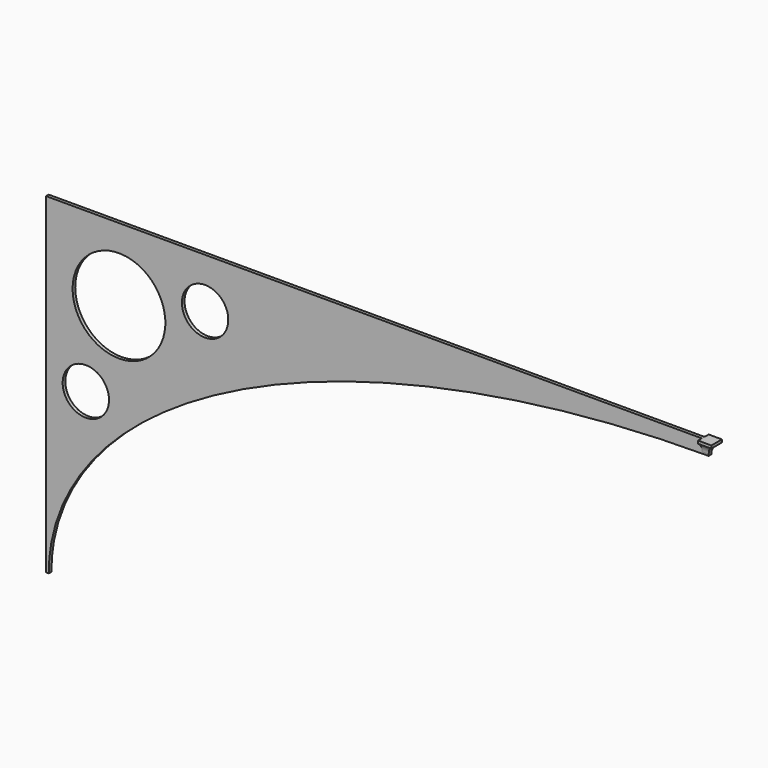
from build123d import *

# Parameters (mm, degrees)
F1_DEPTH     = 2.5
F3_D         = 70
F4_D         = 35
F5_W         = 5
F5_H         = 2.5
F6_DEPTH     = 2
F7_DEPTH     = 0.1
F8_T1_DEPTH  = 2.5
F8_T3_DEPTH  = 5
F8_T9_DEPTH  = 21.0404962177
F8_T14_DEPTH = 21.9443021397
F8_T22_DEPTH = 21.0404962177
F8_T27_DEPTH = 21.9443021397


# Not quite as in the source:
# - a fillet or chamfer that OpenCascade refuses, or shapes differently, is made with other operations: its cross-section is extruded or revolved along the edge and cut away or added


with BuildPart() as f1:
    # F0 (on Front) → F1 (new body)
    with BuildSketch(Plane.XZ):
        with BuildLine():
            Line((234.3109268695, 164.7265180945), (-265.6890731305, 164.7265180945))
            Line((-265.6890731305, 164.7265180945), (-265.6890731305, -85.2734819055))
            Line((-265.6890731305, -85.2734819055), (-263.6890731305, -85.2734819055))
            add(Edge.make_bspline(
                [(234.3109268695, 154.7265180945), (-263.6890731305, 154.7265180945), (-263.6890731305, -85.2734819055)],
                knots=[4.7123889804, 4.7123889804, 4.7123889804, 6.2831853072, 6.2831853072, 6.2831853072], degree=2, weights=[1, 0.7071067812, 1]))
            Line((234.3109268695, 154.7265180945), (234.3109268695, 164.7265180945))
        make_face()
    extrude(amount=F1_DEPTH)

    # F3 (through all)
    with Locations(Plane.XZ.offset(2.5)):
        with Locations((-210.6890731305, 109.7265180945)):
            Hole(F3_D / 2)

    # F4 (through all)
    with Locations(Plane.XZ.offset(2.5)):
        with Locations((-145.6890731305, 127.2265180945), (-235.6890731305, 44.7265180945)):
            Hole(F4_D / 2)

    # F5 (on face) → F6 (join)
    with BuildSketch(Plane.XY.offset(164.7265180945)):
        Polygon((239.3109268695, -6.25), (239.3109268695, 3.75), (229.3109268695, 3.75), (229.3109268695, 0), (234.3109268695, 0), (234.3109268695, -2.5), (229.3109268695, -2.5), (229.3109268695, -6.25), align=None)
        with Locations((231.8109268695, -1.25)):
            Rectangle(F5_W, F5_H)
    extrude(amount=-F6_DEPTH)

    # F5 (on face) → F7 (join)
    with BuildSketch(Plane.XY.offset(164.7265180945)):
        Polygon((239.3109268695, -6.25), (239.3109268695, 3.75), (229.3109268695, 3.75), (229.3109268695, 0), (234.3109268695, 0), (234.3109268695, -2.5), (229.3109268695, -2.5), (229.3109268695, -6.25), align=None)
        with Locations((231.8109268695, -1.25)):
            Rectangle(F5_W, F5_H)
    extrude(amount=F7_DEPTH)

    # F8: fillet of radius 8 on 3 edges, made by hand

    # F8_s2 → F8_t1 (join)
    with BuildSketch(Plane.XZ):
        with BuildLine():
            ThreePointArc((234.3109268695, 155.3103196074), (235.6776772888, 159.7824555624), (239.3109268695, 162.7265180945))
            Line((239.3109268695, 162.7265180945), (234.3109268695, 162.7265180945))
            Line((234.3109268695, 162.7265180945), (234.3109268695, 155.3103196074))
        make_face()
    extrude(amount=F8_T1_DEPTH)

    # F8_s4 → F8_t3 (join)
    with BuildSketch(Plane.YZ.offset(229.3109268695)):
        with BuildLine():
            ThreePointArc((-2.5, 155.9487972387), (-3.5, 159.8217805849), (-6.25, 162.7265180945))
            Line((-6.25, 162.7265180945), (-2.5, 162.7265180945))
            Line((-2.5, 162.7265180945), (-2.5, 155.9487972387))
        make_face()
        with BuildLine():
            ThreePointArc((3.75, 162.7265180945), (1, 159.8217805849), (0, 155.9487972387))
            Line((0, 155.9487972387), (0, 162.7265180945))
            Line((0, 162.7265180945), (3.75, 162.7265180945))
        make_face()
    extrude(amount=F8_T3_DEPTH)


with BuildPart() as f8_tool7:
    # F8_s8 → F8_t9 (new body)
    with BuildSketch(Plane.XZ.offset(21.0404962177)):
        with BuildLine():
            ThreePointArc((234.3109268695, 155.3103196074), (235.6776772888, 159.7824555624), (239.3109268695, 162.7265180945))
            Line((239.3109268695, 162.7265180945), (234.3109268695, 162.7265180945))
            Line((234.3109268695, 162.7265180945), (234.3109268695, 155.3103196074))
        make_face()
    extrude(amount=-F8_T9_DEPTH)

    split(bisect_by=Plane.XZ.offset(6.25), keep=Keep.BOTTOM)

    split(bisect_by=Plane.XZ.offset(2.5), keep=Keep.TOP)


with BuildPart() as f8_tool12:
    # F8_s13 → F8_t14 (new body)
    with BuildSketch(Plane.YZ.offset(251.2552290092)):
        with BuildLine():
            ThreePointArc((-2.5, 155.9487972387), (-3.5, 159.8217805849), (-6.25, 162.7265180945))
            Line((-6.25, 162.7265180945), (-2.5, 162.7265180945))
            Line((-2.5, 162.7265180945), (-2.5, 155.9487972387))
        make_face()
    extrude(amount=-F8_T14_DEPTH)

    split(bisect_by=Plane.YZ.offset(234.3109268695), keep=Keep.TOP)

    split(bisect_by=Plane.YZ.offset(239.3109268695), keep=Keep.BOTTOM)


with BuildPart() as f8_tool7_1:
    add(f8_tool7.part)

    # F8_t17: intersect F8_tool12
    add(f8_tool12.part, mode=Mode.INTERSECT)


with BuildPart() as f1_1:
    add(f1.part)

    # F8_t5: union F8_tool7
    add(f8_tool7_1.part)


with BuildPart() as f8_tool20:
    # F8_s21 → F8_t22 (new body)
    with BuildSketch(Plane.XZ.offset(2.5)):
        with BuildLine():
            ThreePointArc((234.3109268695, 155.3103196074), (235.6776772888, 159.7824555624), (239.3109268695, 162.7265180945))
            Line((239.3109268695, 162.7265180945), (234.3109268695, 162.7265180945))
            Line((234.3109268695, 162.7265180945), (234.3109268695, 155.3103196074))
        make_face()
    extrude(amount=-F8_T22_DEPTH)

    split(bisect_by=Plane.XZ.offset(-3.75), keep=Keep.TOP)

    split(bisect_by=Plane.XZ, keep=Keep.BOTTOM)


with BuildPart() as f8_tool25:
    # F8_s26 → F8_t27 (new body)
    with BuildSketch(Plane.YZ.offset(251.2552290092)):
        with BuildLine():
            ThreePointArc((3.75, 162.7265180945), (1, 159.8217805849), (0, 155.9487972387))
            Line((0, 155.9487972387), (0, 162.7265180945))
            Line((0, 162.7265180945), (3.75, 162.7265180945))
        make_face()
    extrude(amount=-F8_T27_DEPTH)

    split(bisect_by=Plane.YZ.offset(234.3109268695), keep=Keep.TOP)

    split(bisect_by=Plane.YZ.offset(239.3109268695), keep=Keep.BOTTOM)


with BuildPart() as f8_tool20_1:
    add(f8_tool20.part)

    # F8_t30: intersect F8_tool25
    add(f8_tool25.part, mode=Mode.INTERSECT)


with BuildPart() as f1_2:
    add(f1_1.part)

    # F8_t18: union F8_tool20
    add(f8_tool20_1.part)


solid = f1_2.part
